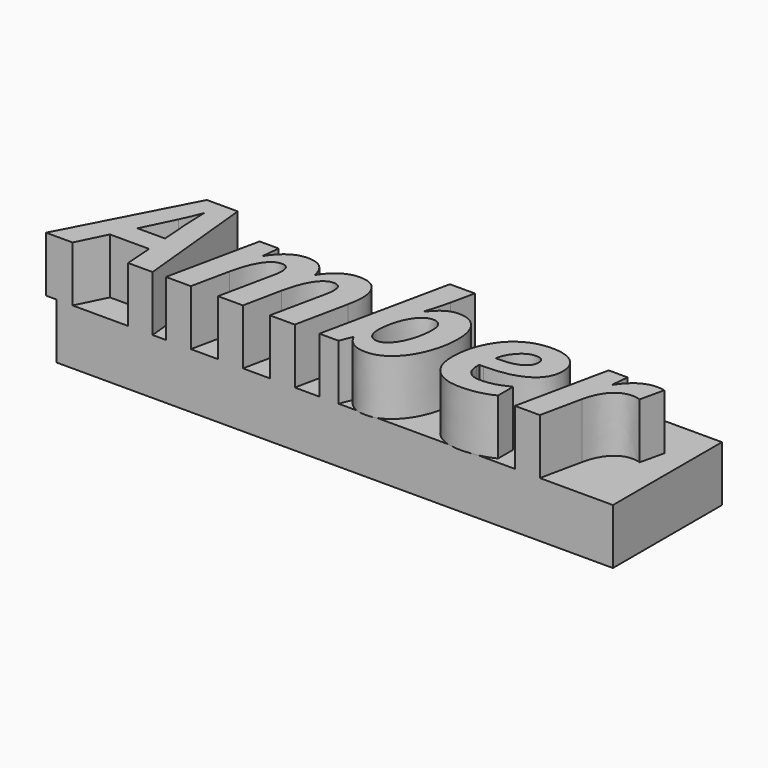
from build123d import *

# Parameters (mm, degrees)
F2_W         = 63.7525618076
F2_H         = 15.6037779525
F3_DEPTH     = 6.35
F0_TEXT_SIZE = 19.431030361
F4_DEPTH     = 6.35


# Not quite as in the source:
# - Text() gives the source's letters only with a copy of the font that has no kerning and outlines rounded to 1/6400 em; it was checked with that copy


with BuildPart() as f3:
    # F2 (on Top) → F3 (new body)
    with BuildSketch(Plane.XY):
        with Locations((31.8762809038, 7.8018889762)):
            Rectangle(F2_W, F2_H)
    extrude(amount=-F3_DEPTH)

    # F0 (on Top) → F4 (join)
    with BuildSketch(Plane.XY):
        with Locations((0, 0)):
            Text('Amber', F0_TEXT_SIZE, font='Open Sans', font_style=FontStyle.BOLDITALIC, text_align=(TextAlign.LEFT, TextAlign.BOTTOM))
    extrude(amount=F4_DEPTH)


solid = f3.part
